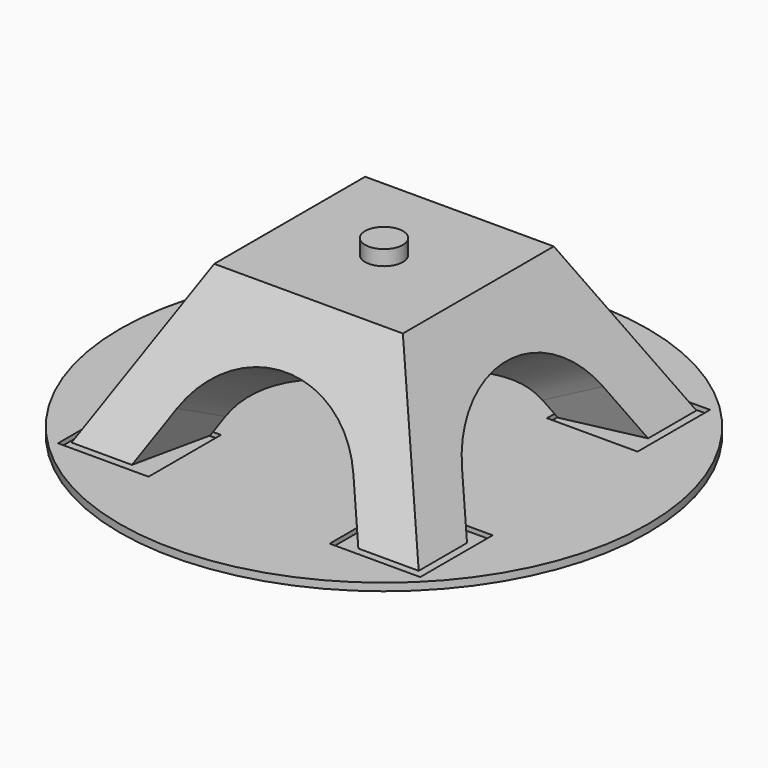
from build123d import *

# Parameters (mm, degrees)
F0_R      = 44.45
F0_R_2    = 3.81
F1_DEPTH  = 1.27
F2_W      = 58.42
F2_H      = 58.42
F4_W      = 31.75
F4_H      = 31.75
F10_DEPTH = 141.478
F11_DEPTH = 70.866
F12_DEPTH = 64.516
F13_DEPTH = 65.278
F14_W     = 15.24
F14_H     = 15.24
F15_DEPTH = 0.762
F16_R     = 3.175
F17_DEPTH = 2.54


with BuildPart() as f1:
    # F0 (on Top) → F1 (new body)
    with BuildSketch(Plane.XY):
        Circle(F0_R)
        Circle(F0_R_2, mode=Mode.SUBTRACT)
    extrude(amount=-F1_DEPTH)

    # F14 (on face) → F15 (cut)
    with BuildSketch(Plane.XY):
        with Locations((-22.86, 22.86)):
            Rectangle(F14_W, F14_H)
        with Locations((22.86, 22.86)):
            Rectangle(F14_W, F14_H)
        with Locations((22.86, -22.86)):
            Rectangle(F14_W, F14_H)
        with Locations((-22.86, -22.86)):
            Rectangle(F14_W, F14_H)
    extrude(amount=-F15_DEPTH, mode=Mode.SUBTRACT)


with BuildPart() as f5:
    # F2 (on Top) → F5 section 0
    with BuildSketch(Plane.XY):
        Rectangle(F2_W, F2_H)
    # F4 (on offset) → F5 section 1
    with BuildSketch(Plane.XY.offset(25.4)):
        Rectangle(F4_W, F4_H)
    loft()

    # F7 (on face) → F10 (cut)
    with BuildSketch(Plane(origin=(-22.8985791279, 0, 12.0217540421), x_dir=(0, -1, 0), z_dir=(-0.8853979028, 0, 0.464833899))):
        with BuildLine():
            Line((-19.05, -13.5777981895), (19.05, -13.5777981895))
            Line((19.05, -13.5777981895), (14.8374191851, -4.5152474072))
            ThreePointArc((14.8374191851, -4.5152474072), (0, 4.9498685856), (-14.8374191851, -4.5152474072))
            Line((-14.8374191851, -4.5152474072), (-19.05, -13.5777981895))
        make_face()
    extrude(amount=-F10_DEPTH, mode=Mode.SUBTRACT)

    # F8 (on face) → F11 (cut)
    with BuildSketch(Plane(origin=(0, -22.8985791279, 12.0217540421), x_dir=(1, 0, 0), z_dir=(0, -0.8853979028, 0.464833899))):
        with BuildLine():
            Line((-14.8374191851, -4.5152474072), (-19.05, -13.5777981895))
            Line((-19.05, -13.5777981895), (19.05, -13.5777981895))
            Line((19.05, -13.5777981895), (14.8374191851, -4.5152474072))
            ThreePointArc((14.8374191851, -4.5152474072), (0, 4.9498685856), (-14.8374191851, -4.5152474072))
        make_face()
    extrude(amount=-F11_DEPTH, mode=Mode.SUBTRACT)

    # F9 (on face) → F12 (cut)
    with BuildSketch(Plane(origin=(22.8985791279, 0, 12.0217540421), x_dir=(0, 1, 0), z_dir=(0.8853979028, 0, 0.464833899))):
        with BuildLine():
            Line((-19.05, -13.5777981895), (19.05, -13.5777981895))
            Line((19.05, -13.5777981895), (14.8374191851, -4.5152474072))
            ThreePointArc((14.8374191851, -4.5152474072), (0, 4.9498685856), (-14.8374191851, -4.5152474072))
            Line((-14.8374191851, -4.5152474072), (-19.05, -13.5777981895))
        make_face()
    extrude(amount=-F12_DEPTH, mode=Mode.SUBTRACT)

    # F6 (on face) → F13 (cut)
    with BuildSketch(Plane(origin=(0, 22.8985791279, 12.0217540421), x_dir=(-1, 0, 0), z_dir=(0, 0.8853979028, 0.464833899))):
        with BuildLine():
            Line((-19.05, -13.5777981895), (19.05, -13.5777981895))
            Line((19.05, -13.5777981895), (14.8374191851, -4.5152474072))
            ThreePointArc((14.8374191851, -4.5152474072), (0, 4.9498685856), (-14.8374191851, -4.5152474072))
            Line((-14.8374191851, -4.5152474072), (-19.05, -13.5777981895))
        make_face()
    extrude(amount=-F13_DEPTH, mode=Mode.SUBTRACT)

    # F16 (on face) → F17 (join)
    with BuildSketch(Plane.XY.offset(25.4)):
        Circle(F16_R)
    extrude(amount=F17_DEPTH)


solid = Compound([f1.part, f5.part])
